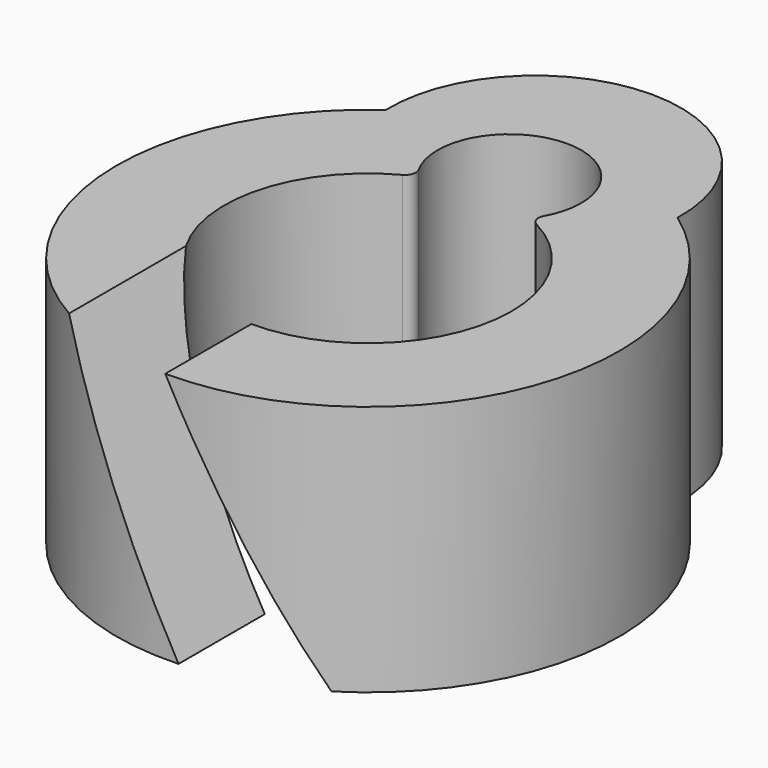
from build123d import *

# Parameters (mm, degrees)
F1_DEPTH = 3.5
F2_R     = 0.15
F4_DEPTH = 25


with BuildPart() as f1:
    # F0 (on Top) → F1 (new body)
    with BuildSketch(Plane.XY):
        with BuildLine():
            ThreePointArc((2.0309193372, 2.850502876), (0, 4.9428488608), (-2.0309193372, 2.850502876))
            ThreePointArc((-2.0309193372, 2.850502876), (0, -3.5), (2.0309193372, 2.850502876))
        make_face()
        with BuildLine():
            ThreePointArc((0.7830913136, 1.8403173625), (0, -2), (-0.7830913136, 1.8403173625))
            ThreePointArc((-0.7830913136, 1.8403173625), (0, 3.4622241035), (0.7830913136, 1.8403173625))
        make_face(mode=Mode.SUBTRACT)
    extrude(amount=F1_DEPTH)

    # F2
    f2_edges = [f1.edges().sort_by_distance(p)[0] for p in [
        (-0.783091, 1.840317, 1.75),
        (0.783091, 1.840317, 1.75),
    ]]
    fillet(f2_edges, radius=F2_R)

    # F3 (on Front) → F4 (cut)
    with BuildSketch(Plane.XZ):
        Polygon((-2.6012919649, 8.286720852), (-4.2398504038, 8.1655834162), (3.1280116344, -5.5110100095), (4.8318293002, -5.5110100095), align=None)
    extrude(amount=F4_DEPTH, mode=Mode.SUBTRACT)


solid = f1.part
